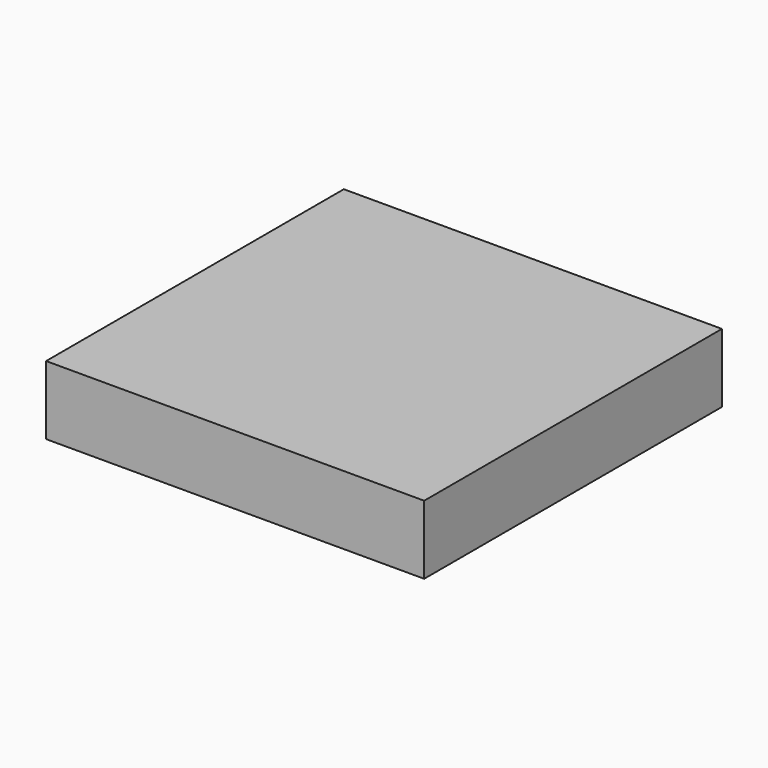
from build123d import *

# Parameters (mm, degrees)
F0_W     = 69.8630958796
F0_H     = 137.5265717506
F3_DEPTH = 25.4


# Not quite as in the source:
# - the program builds the solid bodies; features that only make, move or delete a surface that nothing else refers to are left out


with BuildPart() as f3:
    # F0 (on Top) → F3 (new body)
    with BuildSketch(Plane.XY):
        with Locations((34.9315479398, 0)):
            Rectangle(F0_W, F0_H)
        with Locations((-34.9315479398, 0)):
            Rectangle(F0_W, F0_H)
    extrude(amount=F3_DEPTH)


solid = f3.part
